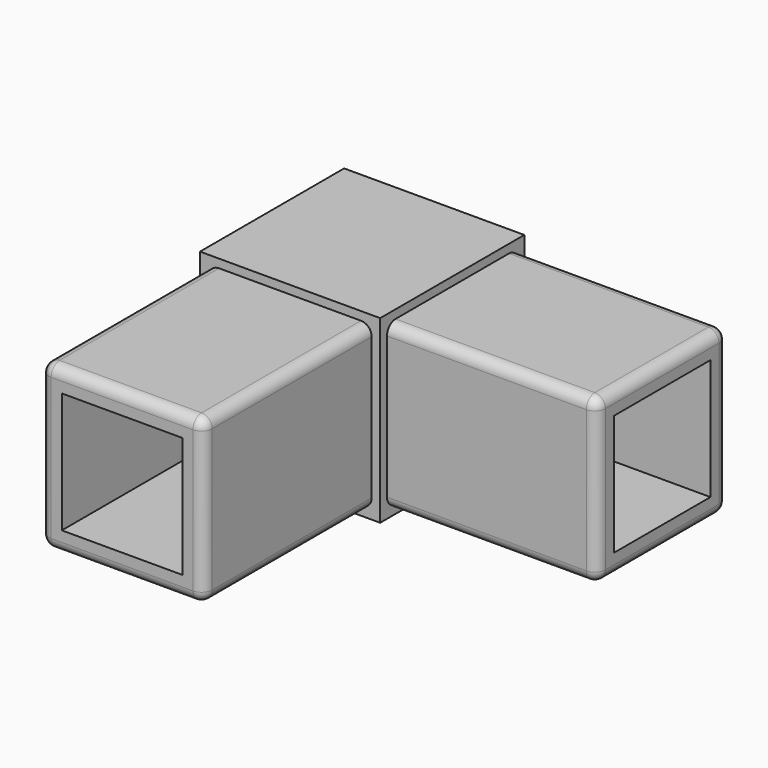
from build123d import *

# Parameters (mm, degrees)
F0_W     = 25.4
F0_H     = 25.4
F1_DEPTH = 12.7
F2_W     = 23
F2_H     = 23
F2_W_2   = 17
F2_H_2   = 17
F3_DEPTH = 29.6
F4_R     = 1.5


# Not quite as in the source:
# - a pattern or mirror of a feature is missing from the dataset's text; its kind, count and spacing are read off the source's solid


with BuildPart() as f1:
    # F0 (on Front) → F1 (new body, symmetric)
    with BuildSketch(Plane.XZ):
        Rectangle(F0_W, F0_H)
    extrude(amount=F1_DEPTH, both=True)

    # F2 (on face) → F3 (join)
    with BuildSketch(Plane.XZ.offset(12.7)):
        Rectangle(F2_W, F2_H)
        Rectangle(F2_W_2, F2_H_2, mode=Mode.SUBTRACT)
    f3 = extrude(amount=F3_DEPTH)

    # F3_copies: F3 across plane
    add(f3.mirror(Plane(origin=(0, 0, 0), x_dir=(-0.7071067812, 0.7071067812, 0), z_dir=(0.7071067812, 0.7071067812, 0))))

    # F4
    f4_edges = [f1.edges().sort_by_distance(p)[0] for p in [
        (11.5, -27.5, 11.5),
        (11.5, -27.5, -11.5),
        (-11.5, -27.5, 11.5),
        (-11.5, -27.5, -11.5),
        (0, -42.3, 11.5),
        (11.5, -42.3, 0),
        (0, -42.3, -11.5),
        (-11.5, -42.3, 0),
        (27.5, -11.5, -11.5),
        (27.5, -11.5, 11.5),
        (42.3, -11.5, 0),
        (27.5, 11.5, -11.5),
        (42.3, 0, -11.5),
        (27.5, 11.5, 11.5),
        (42.3, 11.5, 0),
        (42.3, 0, 11.5),
    ]]
    fillet(f4_edges, radius=F4_R)


solid = f1.part
